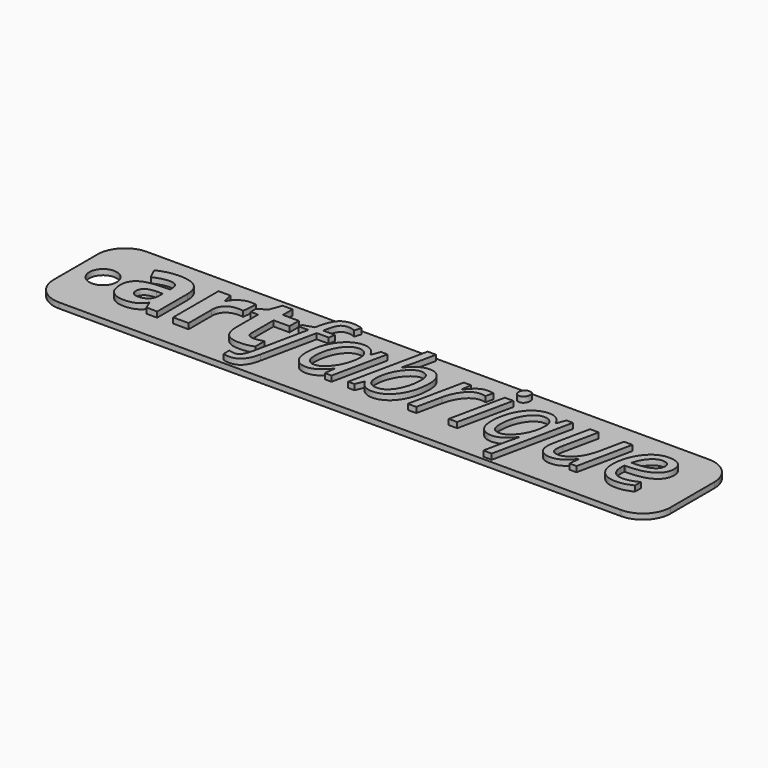
from build123d import *

# Parameters (mm, degrees)
F0_W           = 90
F0_H           = 16
F0_R           = 2
F1_DEPTH       = 0.8
F2_R           = 4
F3_TEXT_SIZE   = 15.1734116824
F3_TEXT_SIZE_2 = 15.0916279785
F4_DEPTH       = 0.8


# Not quite as in the source:
# - Text() gives the source's letters only with a copy of the font that has no kerning and outlines rounded to 1/6400 em; it was checked with that copy


with BuildPart() as f1:
    # F0 (on Top) → F1 (new body)
    with BuildSketch(Plane.XY):
        with Locations((45, 8)):
            Rectangle(F0_W, F0_H)
        with Locations((4, 8)):
            Circle(F0_R, mode=Mode.SUBTRACT)
    extrude(amount=F1_DEPTH)

    # F2
    f2_edges = [f1.edges().sort_by_distance(p)[0] for p in [
        (90, 0, 0.4),
        (90, 16, 0.4),
        (0, 16, 0.4),
        (0, 0, 0.4),
    ]]
    fillet(f2_edges, radius=F2_R)

    # F3 (on face) → F4 (join)
    with BuildSketch(Plane.XY.offset(0.8)):
        with Locations((7.0517212152, 4.0287792217)):
            Text('art', F3_TEXT_SIZE, font='Open Sans', font_style=FontStyle.BOLD, text_align=(TextAlign.LEFT, TextAlign.BOTTOM))
        with Locations((29.2049022715, 4.0876634885)):
            Text('fabrique', F3_TEXT_SIZE_2, font='Open Sans', font_style=FontStyle.ITALIC, text_align=(TextAlign.LEFT, TextAlign.BOTTOM))
    extrude(amount=F4_DEPTH)


solid = f1.part
